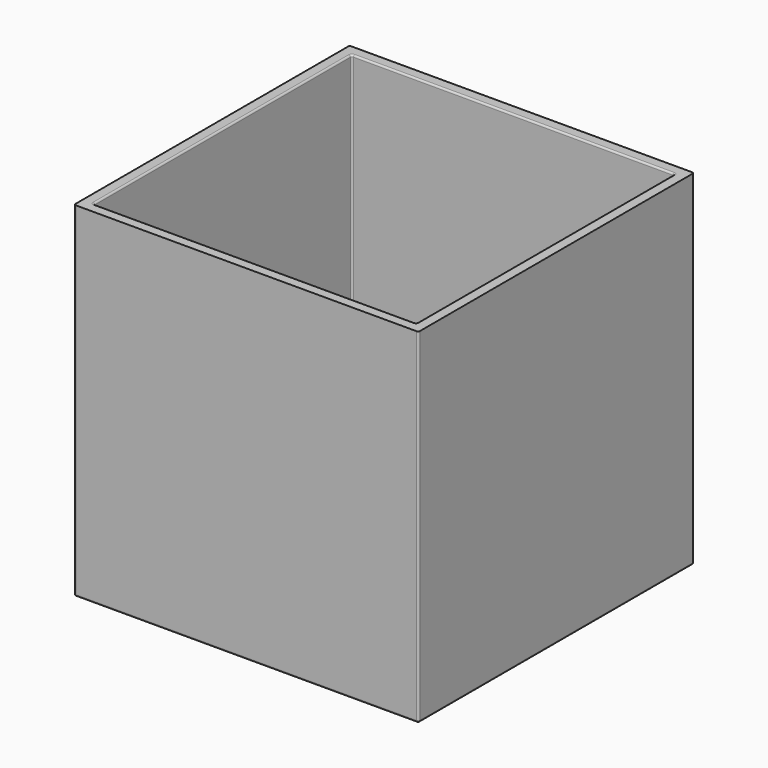
from build123d import *

# Parameters (mm, degrees)
F0_W         = 50.8
F0_H         = 50.8
F1_DEPTH     = 1.5875
F2_W         = 50.8
F2_H         = 50.8
F2_W_2       = 47.625
F2_H_2       = 47.625
F3_DEPTH     = 49.2125
F4_R         = 0.254
F5_TEXT_SIZE = 8.1110825992
F6_DEPTH     = 0.254


# Not quite as in the source:
# - Text() gives the source's letters only with a copy of the font that has no kerning and outlines rounded to 1/6400 em; it was checked with that copy


with BuildPart() as f1:
    # F0 (on Top) → F1 (new body)
    with BuildSketch(Plane.XY):
        Rectangle(F0_W, F0_H)
    extrude(amount=F1_DEPTH)

    # F2 (on face) → F3 (join)
    with BuildSketch(Plane.XY.offset(1.5875)):
        Rectangle(F2_W, F2_H)
        Rectangle(F2_W_2, F2_H_2, mode=Mode.SUBTRACT)
    extrude(amount=F3_DEPTH)

    # F4
    f4_edges = [f1.edges().sort_by_distance(p)[0] for p in [
        (-23.8125, 0, 1.5875),
        (-23.8125, -23.8125, 26.19375),
        (0, -23.8125, 1.5875),
        (-23.8125, 0, 50.8),
        (0, -23.8125, 50.8),
        (0, 23.8125, 1.5875),
        (-23.8125, 23.8125, 26.19375),
        (0, 23.8125, 50.8),
        (23.8125, 23.8125, 26.19375),
        (23.8125, 0, 1.5875),
        (23.8125, 0, 50.8),
        (23.8125, -23.8125, 26.19375),
        (-25.4, -25.4, 25.4),
        (25.4, -25.4, 25.4),
        (25.4, 25.4, 25.4),
        (-25.4, 25.4, 25.4),
        (-25.4, 0, 0),
        (0, -25.4, 0),
        (0, 25.4, 0),
        (25.4, 0, 0),
    ]]
    fillet(f4_edges, radius=F4_R)

    # F5 (on face) → F6 (cut)
    with BuildSketch(Plane(origin=(0, 25.4, 0), x_dir=(-1, 0, 0), z_dir=(0, 1, 0))):
        with Locations((-22.225, 32.2600205286)):
            Text('Powerpoles', F5_TEXT_SIZE, font='Open Sans', text_align=(TextAlign.LEFT, TextAlign.BOTTOM))
    extrude(amount=-F6_DEPTH, mode=Mode.SUBTRACT)


solid = f1.part
